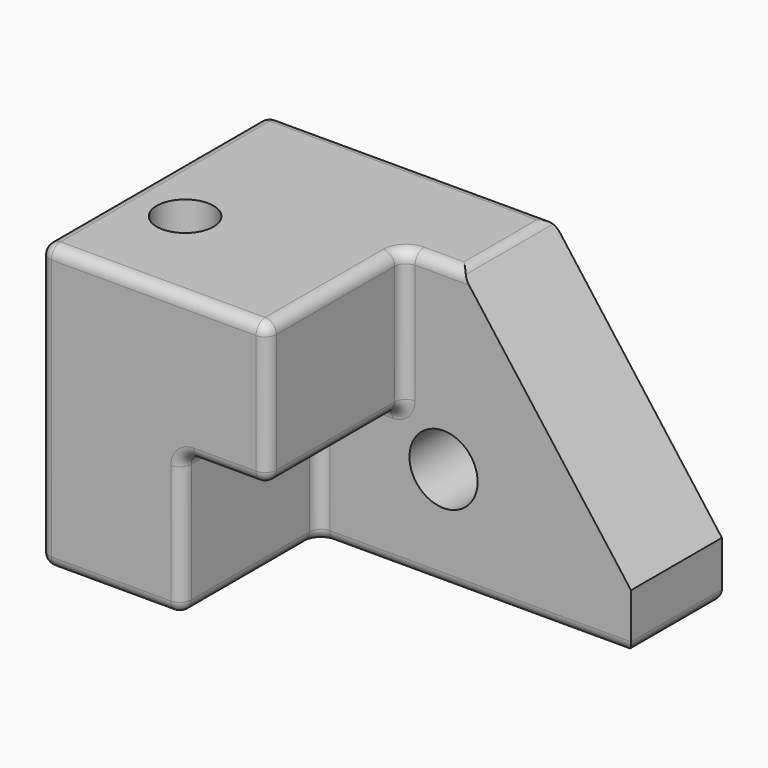
from build123d import *

# Parameters (mm, degrees)
F0_W     = 203.2
F0_H     = 127
F1_DEPTH = 127
F3_DEPTH = 76.2
F4_SIZE2 = 101.6
F4_SIZE  = 76.2
F5_R     = 5.08
F6_R     = 15.24
F7_DEPTH = 50.8
F8_R     = 12.7
F9_DEPTH = 127


with BuildPart() as f1:
    # F0 (on Front) → F1 (new body)
    with BuildSketch(Plane.XZ):
        Rectangle(F0_W, F0_H)
    extrude(amount=F1_DEPTH)

    # F2 (on face) → F3 (cut)
    with BuildSketch(Plane.XZ.offset(127)):
        Polygon((-38.1, 0), (-38.1, -63.5), (101.6, -63.5), (101.6, 63.5), (0, 63.5), (0, 0), align=None)
    extrude(amount=-F3_DEPTH, mode=Mode.SUBTRACT)

    # F4
    f4_edges = [f1.edges().sort_by_distance(p)[0] for p in [
        (101.6, -25.4, 63.5),
    ]]
    f4_side = f1.faces().sort_by_distance((-21.771429, -52.614286, 63.5))[0]
    chamfer(f4_edges, length=F4_SIZE, length2=F4_SIZE2, reference=f4_side)

    # F5
    f5_edges = [f1.edges().sort_by_distance(p)[0] for p in [
        (-50.8, -127, 63.5),
        (0, -88.9, 63.5),
        (0, -50.8, 31.75),
        (25.4, -25.4, 63.5),
        (-38.1, 0, 63.5),
        (-101.6, -63.5, 63.5),
        (0, -127, 31.75),
        (-19.05, -127, 0),
        (0, -88.9, 0),
        (-38.1, -127, -31.75),
        (-38.1, -50.8, -31.75),
        (-38.1, -88.9, -63.5),
        (-69.85, -127, -63.5),
        (-101.6, -127, 0),
        (-38.1, -88.9, 0),
        (-101.6, -63.5, -63.5),
        (0, 0, -63.5),
        (101.6, -25.4, -63.5),
        (-101.6, 0, 0),
        (31.75, -50.8, -63.5),
        (12.7, -50.8, 63.5),
        (-19.05, -50.8, 0),
    ]]
    fillet(f5_edges, radius=F5_R)

    # F6 (on face) → F7 (cut, through all)
    with BuildSketch(Plane.XZ.offset(50.8)):
        with Locations((17.78, -17.78)):
            Circle(F6_R)
    extrude(amount=-F7_DEPTH, mode=Mode.SUBTRACT)

    # F8 (on face) → F9 (cut, through all)
    with BuildSketch(Plane.XY.offset(63.5)):
        with Locations((-74.6759995818, -79.6290040016)):
            Circle(F8_R)
    extrude(amount=-F9_DEPTH, mode=Mode.SUBTRACT)


solid = f1.part
